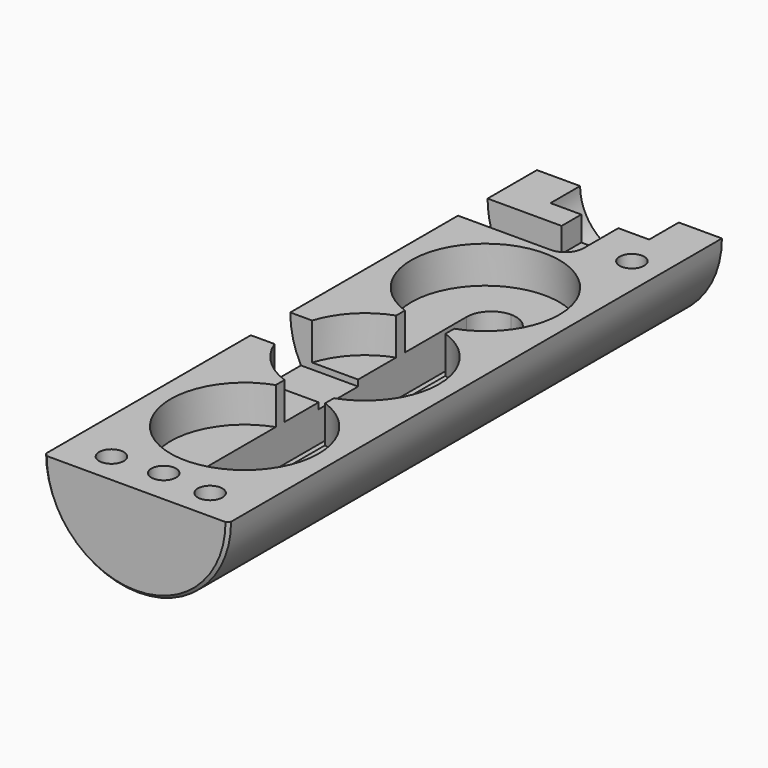
from build123d import *

# Parameters (mm, degrees)
F1_DEPTH  = 50
F2_R      = 6
F3_DEPTH  = 3
F4_R      = 4
F5_DEPTH  = 3
F6_W      = 4
F6_H      = 30
F7_DEPTH  = 6
F8_R      = 1.99999
F9_W      = 9.3910377485
F9_H      = 4
F10_DEPTH = 3.5
F12_D     = 2
F12_DEPTH = 4
F12_TIP   = 0.600860619
F14_DEPTH = 2
F15_R     = 1.5
F16_SIZE  = 0.25
F18_R     = 1
F19_DEPTH = 3
F20_R     = 1
F21_DEPTH = 3


# Not quite as in the source:
# - a fillet or chamfer is up to 0.001 mm smaller than in the source, because OpenCascade refuses the exact size


with BuildPart() as f1:
    # F0 (on Front) → F1 (new body)
    with BuildSketch(Plane.XZ):
        with BuildLine():
            Line((7.5, 0), (-7.5, 0))
            ThreePointArc((-7.5, 0), (0, -7.5), (7.5, 0))
        make_face()
    extrude(amount=F1_DEPTH)

    # F2 (on face) → F3 (cut)
    with BuildSketch(Plane.XY):
        with Locations((0, -39)):
            Circle(F2_R)
        with Locations((0, -26.8)):
            Circle(F2_R)
        with Locations((0, -14.6)):
            Circle(F2_R)
    extrude(amount=-F3_DEPTH, mode=Mode.SUBTRACT)

    # F4 (on face) → F5 (cut)
    with BuildSketch(Plane(origin=(0, 0, 0), x_dir=(-1, 0, 0), z_dir=(0, 1, 0))):
        Circle(F4_R)
    extrude(amount=-F5_DEPTH, mode=Mode.SUBTRACT)

    # F6 (on face) → F7 (cut)
    with BuildSketch(Plane.XY):
        with Locations((0, -27)):
            Rectangle(F6_W, F6_H)
    extrude(amount=-F7_DEPTH, mode=Mode.SUBTRACT)

    # F8 (radius 2 in the source; OpenCascade refuses exactly that, so slightly less here)
    f8_edges = [f1.edges().sort_by_distance(p)[0] for p in [
        (-2, -12, -4.5),
        (2, -12, -4.5),
        (-2, -42, -4.5),
        (2, -42, -4.5),
    ]]
    fillet(f8_edges, radius=F8_R)

    # F9 (on face) → F10 (cut)
    with BuildSketch(Plane.XY):
        with Locations((-4.6955188743, -27)):
            Rectangle(F9_W, F9_H)
    extrude(amount=-F10_DEPTH, mode=Mode.SUBTRACT)

    # F12
    with Locations(Plane.XY):
        with Locations((5, -6), (0, -47.2)):
            Hole(F12_D / 2, depth=F12_DEPTH)
            with Locations((0, 0, -(F12_DEPTH + F12_TIP / 2))):  # 118° drill point
                Cone(0, F12_D / 2, F12_TIP, mode=Mode.SUBTRACT)

    # F13 (on face) → F14 (cut)
    with BuildSketch(Plane.XY):
        Polygon((1.5, -3), (-1.5, -3), (-1.5, -5), (-8.88405554, -5), (-8.88405554, -8), (-1.5, -8), (1.5, -8), align=None)
    extrude(amount=-F14_DEPTH, mode=Mode.SUBTRACT)

    # F15
    f15_edges = [f1.edges().sort_by_distance(p)[0] for p in [
        (1.5, -8, -1),
    ]]
    fillet(f15_edges, radius=F15_R)

    # F16
    f16_edges = [f1.edges().sort_by_distance(p)[0] for p in [
        (0, -50, -7.5),
    ]]
    chamfer(f16_edges, length=F16_SIZE)

    # F18 (on offset) → F19 (cut)
    with BuildSketch(Plane.YZ.offset(-7.5)):
        with Locations((-3, -2)):
            Circle(F18_R)
        with Locations((-35, -4)):
            Circle(F18_R)
    extrude(amount=F19_DEPTH, mode=Mode.SUBTRACT)

    # F20 (on face) → F21 (cut)
    with BuildSketch(Plane.XY):
        with Locations((-4, -47.5)):
            Circle(F20_R)
        with Locations((4, -47.5)):
            Circle(F20_R)
    extrude(amount=-F21_DEPTH, mode=Mode.SUBTRACT)


solid = f1.part
